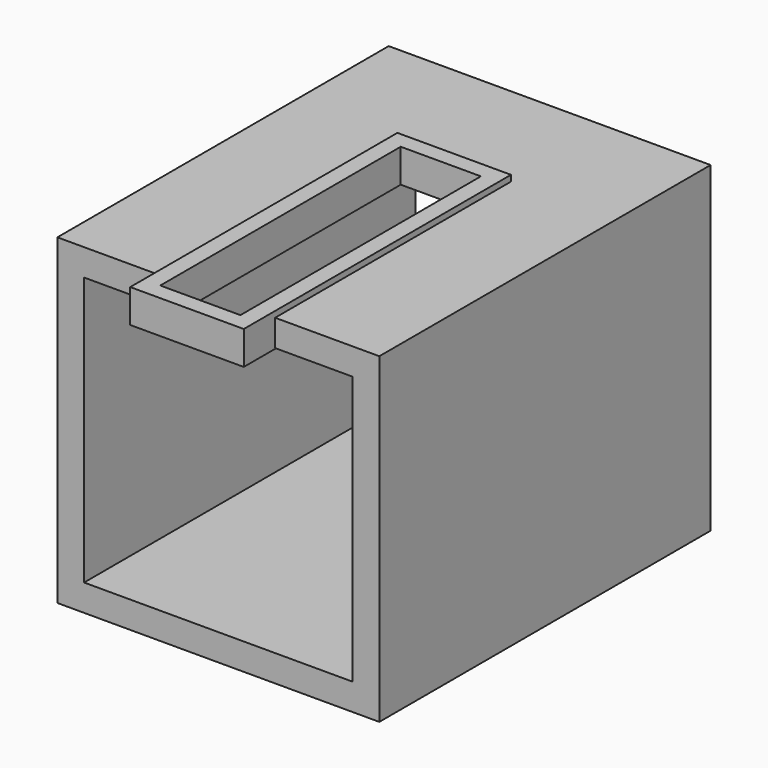
from build123d import *

# Parameters (mm, degrees)
F0_W        = 48.2
F0_H        = 48.2
F0_W_2      = 40.2
F0_H_2      = 40.2
F1_DEPTH    = 62
F3_START    = 20
F2_W        = 17
F2_H        = 50
F3_DEPTH    = 5
F4_T        = 2.5
F4_T3_DEPTH = 49.1321159601
F4_T5_DEPTH = 22
F4_T7_DEPTH = 9
F4_T9_DEPTH = 67


# Not quite as in the source:
# - a shell that OpenCascade refuses in one call is made with other operations: the cavity is built on its own and cut out


with BuildPart() as f1:
    # F0 (on Front) → F1 (new body)
    with BuildSketch(Plane.XZ):
        Rectangle(F0_W, F0_H)
        Rectangle(F0_W_2, F0_H_2, mode=Mode.SUBTRACT)
    extrude(amount=F1_DEPTH)

    # F2 (on Top) → F3 (join)
    with BuildSketch(Plane.XY.offset(F3_START)):
        with Locations((0, -42.8678840399)):
            Rectangle(F2_W, F2_H)
    extrude(amount=F3_DEPTH)

    # F4: shell of thickness 2.5, made by hand


with BuildPart() as f4_core1:
    # F4_t2: copy of F1
    add(f1.part)

    # the walls: a layer under each face that stays
    f4_faces = [f4_core1.faces().sort_by_distance(p)[0] for p in [
        (24.1, -31, 0),
        (0, -31, -24.1),
        (16.0666666667, -51.6666666667, 24.1),
        (-20.6571428571, 0, -20.6571428571),
        (-20.6571428571, -62, -20.6571428571),
        (-24.1, -31, 0),
        (-8.5, -26.2012173732, 24.1666666667),
        (0, -17.8678840399, 24.55),
        (8.5, -59.5345507065, 24.1666666667),
        (20.1, -31, 0),
        (0, -31, -20.1),
        (-20.1, -31, 0),
        (-13.4, -51.6666666667, 20.1),
        (0, -67.8678840399, 22.5),
        (0, -17.8678840399, 20.05),
    ]]
    thicken(f4_faces, amount=-F4_T, mode=Mode.SUBTRACT)

    # F4_s4 → F4_t3 (cut)
    with BuildSketch(Plane.XZ.offset(15.3678840399)):
        Polygon((-8.525, 24.125), (-8.5, 21.6), (-6, 21.6), (-6, 24.1), align=None)
        Polygon((8.525, 24.125), (8.5, 21.6), (6, 21.6), (6, 24.1), align=None)
        Polygon((-8.525, 20.075), (-6, 20.1), (-6, 22.6), (-8.5, 22.6), align=None)
        Polygon((8.525, 20.075), (6, 20.1), (6, 22.6), (8.5, 22.6), align=None)
    extrude(amount=F4_T3_DEPTH, mode=Mode.SUBTRACT)

    # F4_s6 → F4_t5 (cut)
    with BuildSketch(Plane.YZ.offset(-11)):
        Polygon((-17.8428840399, 24.125), (-17.8678840399, 21.6), (-20.3678840399, 21.6), (-20.3678840399, 24.1), align=None)
        Polygon((-17.8428840399, 20.075), (-17.8678840399, 22.6), (-20.3678840399, 22.6), (-20.3678840399, 20.1), align=None)
    extrude(amount=F4_T5_DEPTH, mode=Mode.SUBTRACT)

    # F4_s8 → F4_t7 (cut)
    with BuildSketch(Plane.XY.offset(17.6)):
        Polygon((-8.525, -62.025), (-8.5, -59.5), (-6, -59.5), (-6, -62), align=None)
        Polygon((8.525, -62.025), (8.5, -59.5), (6, -59.5), (6, -62), align=None)
    extrude(amount=F4_T7_DEPTH, mode=Mode.SUBTRACT)

    # F4_s10 → F4_t9 (cut)
    with BuildSketch(Plane.XZ.offset(-2.5)):
        Polygon((20.075, 20.075), (22.6, 20.1), (22.6, 22.6), (20.1, 22.6), align=None)
        Polygon((20.075, -20.075), (22.6, -20.1), (22.6, -22.6), (20.1, -22.6), align=None)
        Polygon((-20.075, -20.075), (-20.1, -22.6), (-22.6, -22.6), (-22.6, -20.1), align=None)
        Polygon((-20.075, 20.075), (-22.6, 20.1), (-22.6, 22.6), (-20.1, 22.6), align=None)
    extrude(amount=F4_T9_DEPTH, mode=Mode.SUBTRACT)


with BuildPart() as f1_1:
    add(f1.part)

    # what is left inside the walls is the cavity
    f4_cavity = [f4_core1.part.solids().sort_by_distance(p)[0] for p in [
        (0, -50.367884, 20.025),
    ]]
    add(f4_cavity, mode=Mode.SUBTRACT)


solid = f1_1.part
